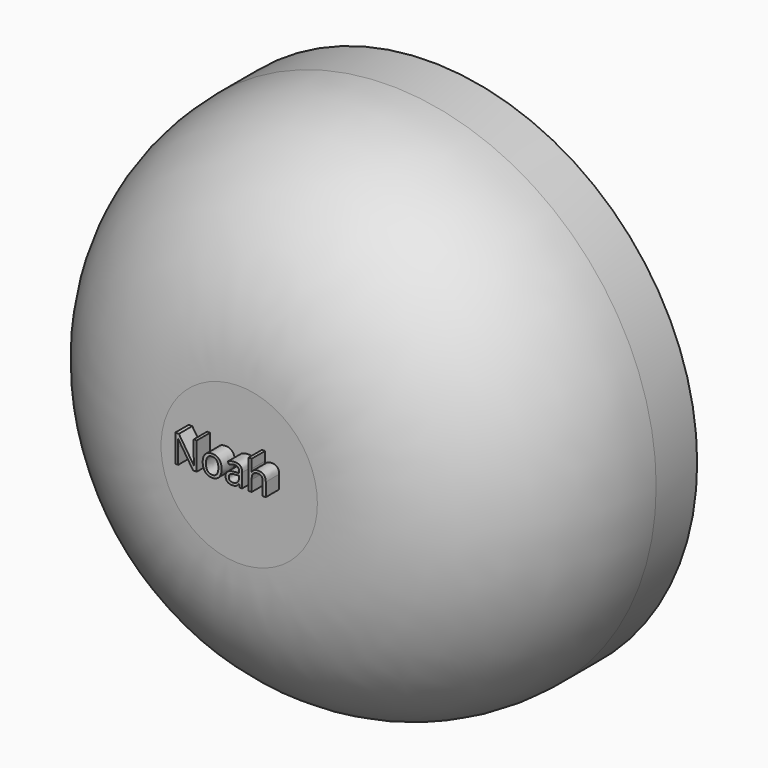
from build123d import *

# Parameters (mm, degrees)
F0_R         = 36.4530048289
F1_DEPTH     = 32.766
F2_R         = 25.7548302834
F3_T         = -2.54
F4_TEXT_SIZE = 5.2715845716
F5_DEPTH     = 35.052


# Not quite as in the source:
# - Text() gives the source's letters only with a copy of the font that has no kerning and outlines rounded to 1/6400 em; it was checked with that copy


with BuildPart() as f1:
    # F0 (on Front) → F1 (new body)
    with BuildSketch(Plane.XZ):
        Circle(F0_R)
    extrude(amount=F1_DEPTH)

    # F2
    f2_edges = [f1.edges().sort_by_distance(p)[0] for p in [
        (-36.453005, -32.766, 0),
    ]]
    fillet(f2_edges, radius=F2_R)

    # F3
    f3_openings = [f1.faces().sort_by_distance(p)[0] for p in [
        (0, 0, 0),
    ]]
    offset(amount=F3_T, openings=f3_openings)

    # F4 (on Front) → F5 (join)
    with BuildSketch(Plane.XZ):
        with Locations((-7.439260371, 0)):
            Text('Noah', F4_TEXT_SIZE, font='Open Sans', text_align=(TextAlign.LEFT, TextAlign.BOTTOM))
    extrude(amount=F5_DEPTH)


solid = f1.part
